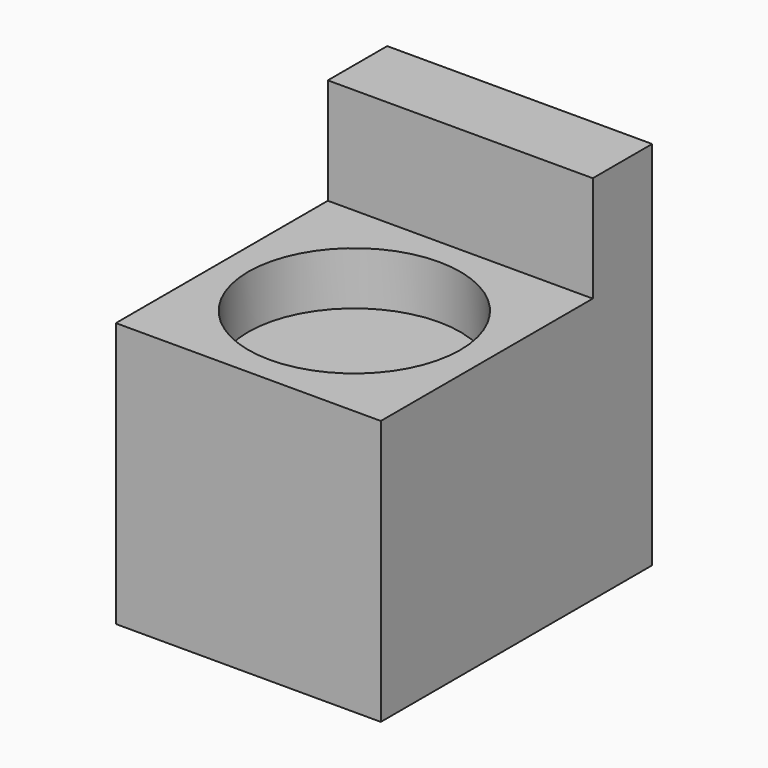
from build123d import *

# Parameters (mm, degrees)
F0_W        = 7
F0_H        = 10
F1_DEPTH    = 25
F2_R        = 10
F3_DEPTH    = 5
F4_T        = 2.5
F4_T3_DEPTH = 30


# Not quite as in the source:
# - a shell that OpenCascade refuses in one call is made with other operations: the cavity is built on its own and cut out


with BuildPart() as f1:
    # F0 (on Right) → F1 (new body)
    with BuildSketch(Plane.YZ):
        with Locations((-3.5, 30)):
            Rectangle(F0_W, F0_H)
        Polygon((-32, 0), (0, 0), (0, 25), (-7, 25), (-32, 25), align=None)
    extrude(amount=F1_DEPTH)

    # F2 (on face) → F3 (cut)
    with BuildSketch(Plane.XY.offset(25)):
        with Locations((12.5, -19.5)):
            Circle(F2_R)
    extrude(amount=-F3_DEPTH, mode=Mode.SUBTRACT)

    # F4: shell of thickness 2.5, made by hand


with BuildPart() as f4_core1:
    # F4_t2: copy of F1
    add(f1.part)

    # the walls: a layer under each face that stays
    f4_faces = [f4_core1.faces().sort_by_distance(p)[0] for p in [
        (12.5, -3.5, 35),
        (12.5, 0, 17.5),
        (12.5, -7, 30),
        (0, -16, 17.5),
        (25, -16, 17.5),
        (20.8333333333, -11.1666666667, 25),
        (12.5, -32, 12.5),
        (2.5, -19.5, 22.5),
        (12.5, -19.5, 20),
    ]]
    thicken(f4_faces, amount=-F4_T, mode=Mode.SUBTRACT)

    # F4_s4 → F4_t3 (cut)
    with BuildSketch(Plane.YZ.offset(-2.5)):
        Polygon((-7.025, 25.025), (-4.5, 25), (-4.5, 22.5), (-7, 22.5), align=None)
    extrude(amount=F4_T3_DEPTH, mode=Mode.SUBTRACT)

    # F4_s5 → F4_t6 (revolve, cut)
    with BuildSketch(Plane.XZ.offset(19.5)):
        Polygon((22.475, 20.025), (25, 20), (25, 17.5), (22.5, 17.5), align=None)
    revolve(axis=Axis((12.5, -19.5, 20), (0, 0, 1)), mode=Mode.SUBTRACT)


with BuildPart() as f1_1:
    add(f1.part)

    # what is left inside the walls is the cavity
    f4_cavity = [f4_core1.part.solids().sort_by_distance(p)[0] for p in [
        (15.833333, -2.525, 16.25),
    ]]
    add(f4_cavity, mode=Mode.SUBTRACT)


solid = f1_1.part
